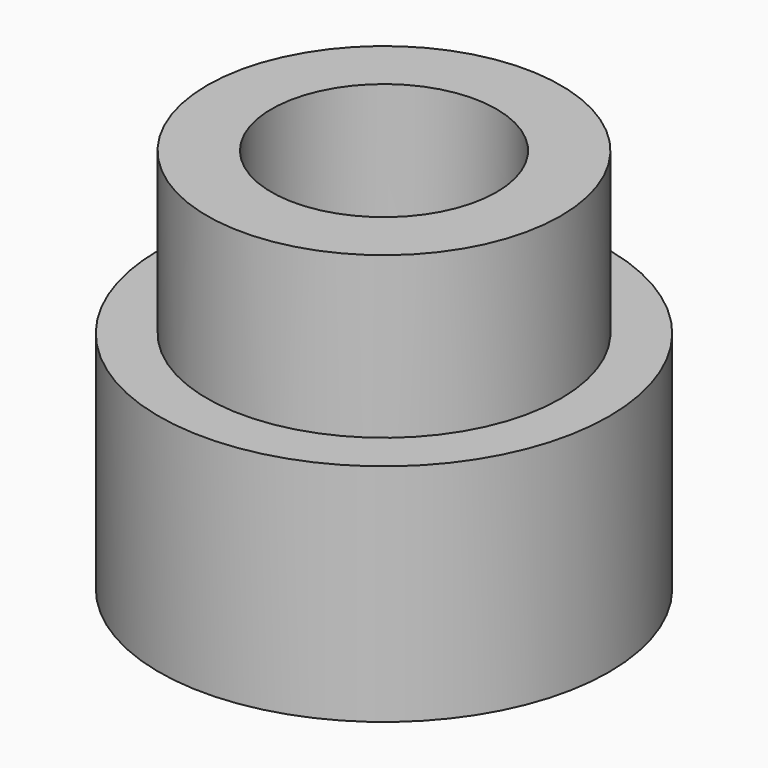
from build123d import *

# Parameters (mm, degrees)
F0_R     = 2.75
F0_R_2   = 1.75
F1_DEPTH = 6
F0_R_3   = 3.5
F2_DEPTH = 3.5


# Not quite as in the source:
# - a feature names something its author has since deleted; it is built from what else it names


with BuildPart() as f1:
    # F0 (on Top) → F1 (new body)
    with BuildSketch(Plane.XY):
        Circle(F0_R)
        Circle(F0_R_2, mode=Mode.SUBTRACT)
    extrude(amount=F1_DEPTH)

    # F0 (on Top) → F2 (join)
    with BuildSketch(Plane.XY):
        Circle(F0_R_3)
        Circle(F0_R, mode=Mode.SUBTRACT)
    extrude(amount=F2_DEPTH)


solid = f1.part
